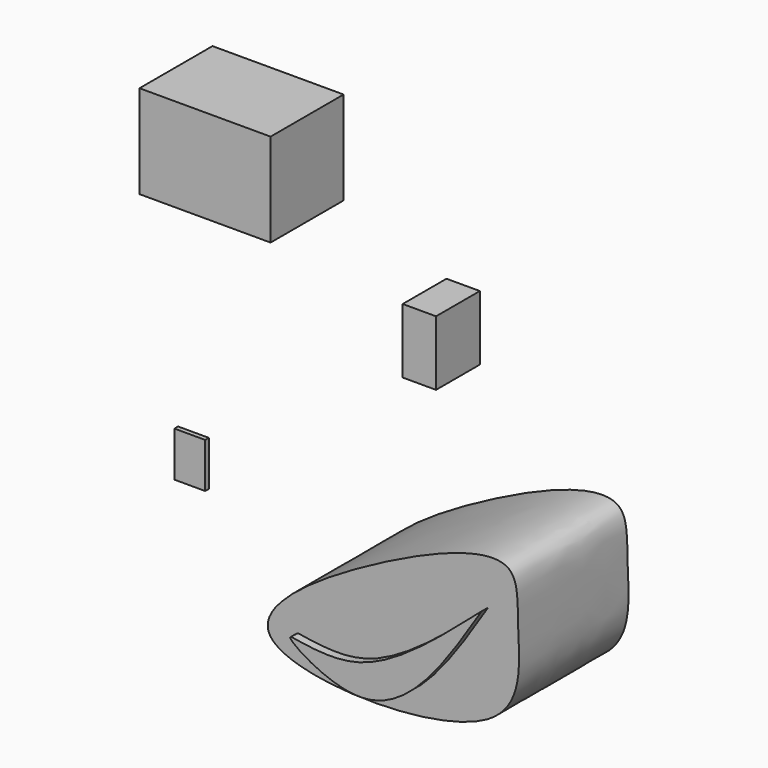
from build123d import *

# Parameters (mm, degrees)
F1_DEPTH  = 30
F2_W      = 28.7323128432
F2_H      = 20.4472616315
F3_DEPTH  = 20
F4_W      = 7.3102321476
F4_H      = 14.1971670091
F5_DEPTH  = 12
F6_W      = 6.7479042336
F6_H      = 9.8608862609
F7_DEPTH  = 1
F12_DEPTH = 1.8


# Not quite as in the source:
# - the program builds the solid bodies; features that only make, move or delete a surface that nothing else refers to are left out


with BuildPart() as f1:
    # F0 (on Front) → F1 (new body)
    with BuildSketch(Plane.XZ):
        with BuildLine():
            add(Edge.make_bspline(
                [(0, -6.7537389696), (4.6302731937, -13.4867750862), (57.4556467963, -14.6892854363), (53.6464783261, 12.0488052166), (54.9550616853, 28.5506433284), (24.9504990775, 17.5929765935), (-3.8399352956, -1.1699597951), (0, -6.7537389696)],
                knots=[0, 0, 0, 0, 0.2678904064, 0.4437728792, 0.5709352547, 0.7778356084, 1, 1, 1, 1], degree=3))
        make_face()
    extrude(amount=-F1_DEPTH)

    # F11 (on face) → F12 (join)
    with BuildSketch(Plane.XZ):
        with BuildLine():
            add(Edge.make_bspline(
                [(47.7026514709, 14.3687073141), (39.7348380228, 1.8481294782), (26.3590902699, -19.1704463134), (4.6243785504, -4.4828704433), (5.8864211069, -4.1930439331), (6.0512563214, -4.1551897302)],
                knots=[0, 0, 0, 0, 0.5615806693, 0.9427381081, 1, 1, 1, 1], degree=3))
            add(Edge.make_bspline(
                [(47.7026514709, 14.3687073141), (38.6932003586, 6.4997414698), (23.3521508086, -6.8993206285), (11.1056602211, -4.956879257), (6.0512563214, -4.1551897302)],
                knots=[0, 0, 0, 0, 0.5872773621, 1, 1, 1, 1], degree=3))
        make_face()
    extrude(amount=F12_DEPTH)


with BuildPart() as f3:
    # F2 (on Front) → F3 (new body)
    with BuildSketch(Plane.XZ):
        with Locations((-14.3661564216, 79.4941745698)):
            Rectangle(F2_W, F2_H)
    extrude(amount=-F3_DEPTH)


with BuildPart() as f5:
    # F4 (on Front) → F5 (new body)
    with BuildSketch(Plane.XZ):
        with Locations((32.6148914173, 59.7432572395)):
            Rectangle(F4_W, F4_H)
    extrude(amount=-F5_DEPTH)


with BuildPart() as f7:
    # F6 (on Front) → F7 (new body)
    with BuildSketch(Plane.XZ):
        with Locations((-17.7132585086, 21.5970976278)):
            Rectangle(F6_W, F6_H)
    extrude(amount=-F7_DEPTH)


solid = Compound([f1.part, f3.part, f5.part, f7.part])
